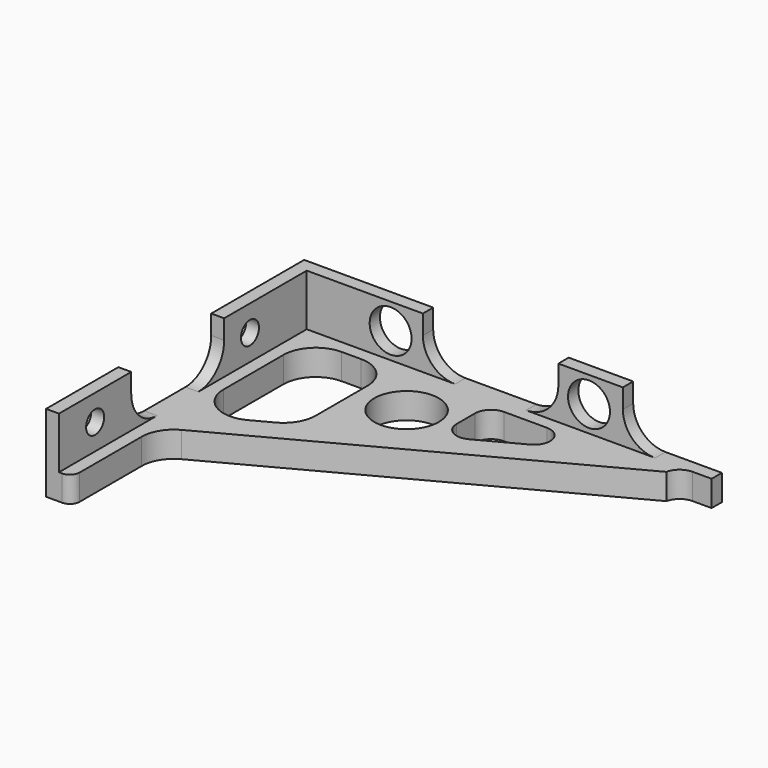
from build123d import *

# Parameters (mm, degrees)
F0_R        = 5
F1_DEPTH    = 4
F2_W        = 10
F2_H        = 2
F2_W_2      = 18
F2_W_3      = 2
F2_H_2      = 14
F3_DEPTH    = 12
F4_R        = 5
F5_T1_DEPTH = 4
F6_R        = 1.5
F7_R        = 3.25
F9_DEPTH    = 2
F8_R        = 1.75
F10_DEPTH   = 2


# Not quite as in the source:
# - a fillet or chamfer that OpenCascade refuses, or shapes differently, is made with other operations: its cross-section is extruded or revolved along the edge and cut away or added


with BuildPart() as f1:
    # F0 (on Top) → F1 (new body)
    with BuildSketch(Plane.XY):
        Polygon((-24.0443362383, -18.3656413368), (31.299512524, 11.1093264446), (31.299512524, 13.1093264446), (36.7056637617, 13.1093264446), (36.7056637617, 15.1093264446), (-28.0443362383, 15.1093264446), (-28.0443362383, -34.8906735554), (-24.0443362383, -34.8906735554), align=None)
        Polygon((-24.0443362383, -13.8337272738), (-24.0443362383, 11.1093264446), (-11.0443362383, 11.1093264446), (3.6275881428, 11.1093264446), (22.7901370984, 11.1093264446), (3.6275881428, 0.9037566169), (-11.0443362383, -6.9102011778), align=None, mode=Mode.SUBTRACT)
        Polygon((3.6275881428, 11.1093264446), (-11.0443362383, 11.1093264446), (-11.0443362383, -6.9102011778), (3.6275881428, 0.9037566169), align=None)
        with Locations((-3.3724118572, 4.1093264446)):
            Circle(F0_R, mode=Mode.SUBTRACT)
    extrude(amount=F1_DEPTH)

    # F2 (on Top) → F3 (join)
    with BuildSketch(Plane.XY):
        with Locations((17.9556637617, 14.1093264446)):
            Rectangle(F2_W, F2_H)
        with Locations((-17.0443362383, 14.1093264446)):
            Rectangle(F2_W_2, F2_H)
        Polygon((-26.0443362383, 15.1093264446), (-28.0443362383, 15.1093264446), (-28.0443362383, -2.8906735554), (-26.0443362383, -2.8906735554), (-26.0443362383, 13.1093264446), align=None)
        with Locations((-27.0443362383, -27.8906735554)):
            Rectangle(F2_W_3, F2_H_2)
    extrude(amount=F3_DEPTH)

    # F4
    f4_edges = [f1.edges().sort_by_distance(p)[0] for p in [
        (-24.044336, 11.109326, 2),
        (-24.044336, -13.833727, 2),
        (-11.044336, -6.910201, 2),
        (-11.044336, 11.109326, 2),
        (-24.044336, -18.365641, 2),
        (-27.044336, -2.890674, 4),
        (-27.044336, -20.890674, 4),
        (-8.044336, 14.109326, 4),
        (12.955664, 14.109326, 4),
        (22.955664, 14.109326, 4),
    ]]
    fillet(f4_edges, radius=F4_R)

    # F5: fillet of radius 2.5 on 4 edges, made by hand

    # F5_s2 → F5_t1 (join)
    with BuildSketch(Plane.XY):
        with BuildLine():
            ThreePointArc((31.299512524, 11.1093264446), (32.1678634367, 12.5458181177), (33.7490022668, 13.1093264446))
            Line((33.7490022668, 13.1093264446), (31.299512524, 13.1093264446))
            Line((31.299512524, 13.1093264446), (31.299512524, 11.1093264446))
        make_face()
        with BuildLine():
            ThreePointArc((6.1275881428, 11.1093264446), (4.3598211899, 10.3770933976), (3.6275881428, 8.6093264446))
            Line((3.6275881428, 8.6093264446), (3.6275881428, 11.1093264446))
            Line((3.6275881428, 11.1093264446), (6.1275881428, 11.1093264446))
        make_face()
        with BuildLine():
            ThreePointArc((7.302762524, 2.8610770581), (4.840719065, 2.9242958576), (3.6275881428, 5.0676502325))
            Line((3.6275881428, 5.0676502325), (3.6275881428, 0.9037566169))
            Line((3.6275881428, 0.9037566169), (7.302762524, 2.8610770581))
        make_face()
        with BuildLine():
            ThreePointArc((12.7776375713, 11.1093264446), (15.2031718358, 9.2149530062), (13.9528119525, 6.4027532703))
            Line((13.9528119525, 6.4027532703), (22.7901370984, 11.1093264446))
            Line((22.7901370984, 11.1093264446), (12.7776375713, 11.1093264446))
        make_face()
    extrude(amount=F5_T1_DEPTH)

    # F6
    f6_edges = [f1.edges().sort_by_distance(p)[0] for p in [
        (-24.044336, -34.890674, 2),
    ]]
    fillet(f6_edges, radius=F6_R)

    # F7 (on face) → F9 (cut)
    with BuildSketch(Plane(origin=(0, 15.1093264446, 0), x_dir=(-1, 0, 0), z_dir=(0, 1, 0))):
        with Locations((-17.7056637617, 8)):
            Circle(F7_R)
        with Locations((13.0443362383, 8)):
            Circle(F7_R)
    extrude(amount=-F9_DEPTH, mode=Mode.SUBTRACT)

    # F8 (on face) → F10 (cut)
    with BuildSketch(Plane(origin=(-28.0443362383, 0, 0), x_dir=(0, -1, 0), z_dir=(-1, 0, 0))):
        with Locations((-2.1093264446, 8)):
            Circle(F8_R)
        with Locations((27.8906735554, 8)):
            Circle(F8_R)
    extrude(amount=-F10_DEPTH, mode=Mode.SUBTRACT)


solid = f1.part
